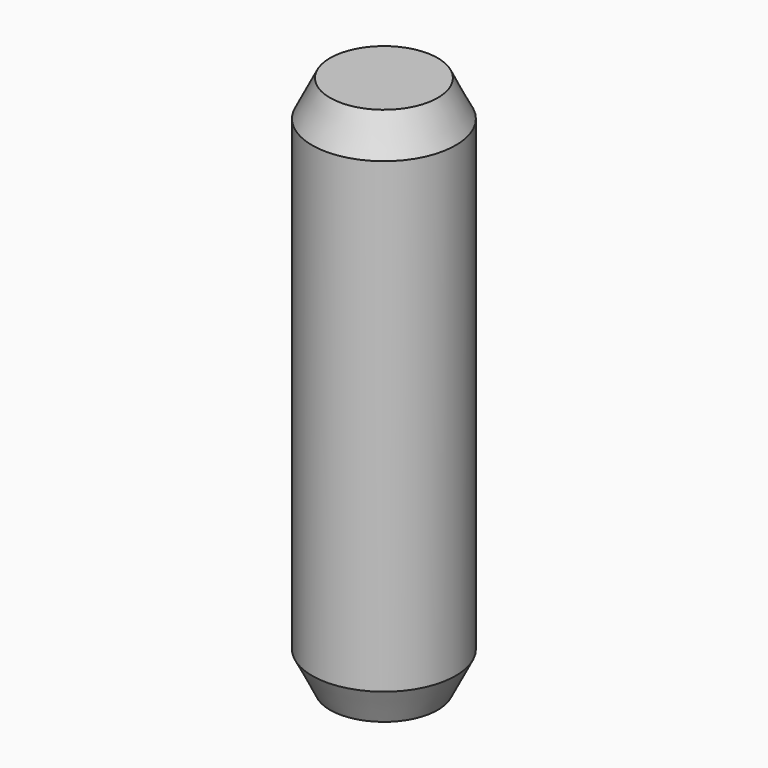
from build123d import *

# Parameters (mm, degrees)
F0_W        = 4
F0_H        = 30
F2_C1_SIZE2 = 2
F2_C1_SIZE  = 1
F2_C2_SIZE2 = 1
F2_C2_SIZE  = 2


# Not quite as in the source:
# - two fillets or chamfers of one size are made in one step


with BuildPart() as f1:
    # F0 (on Front) → F1 (revolve)
    with BuildSketch(Plane.XZ):
        with Locations((-2, 15)):
            Rectangle(F0_W, F0_H)
    revolve(axis=Axis((0, 0, 22.5), (0, 0, 1)))

    # F2: chamfer of 2 x 1 on 2 edges, made by hand

    # F2_c1
    f2_c1_edges = [f1.edges().sort_by_distance(p)[0] for p in [
        (4, 0, 0),
    ]]
    f2_c1_side = f1.faces().sort_by_distance((3.98, 0, 0))[0]
    chamfer(f2_c1_edges, length=F2_C1_SIZE, length2=F2_C1_SIZE2, reference=f2_c1_side)

    # F2_c2
    f2_c2_edges = [f1.edges().sort_by_distance(p)[0] for p in [
        (4, 0, 30),
    ]]
    f2_c2_side = f1.faces().sort_by_distance((4, 0, 29.98))[0]
    chamfer(f2_c2_edges, length=F2_C2_SIZE, length2=F2_C2_SIZE2, reference=f2_c2_side)


solid = f1.part
